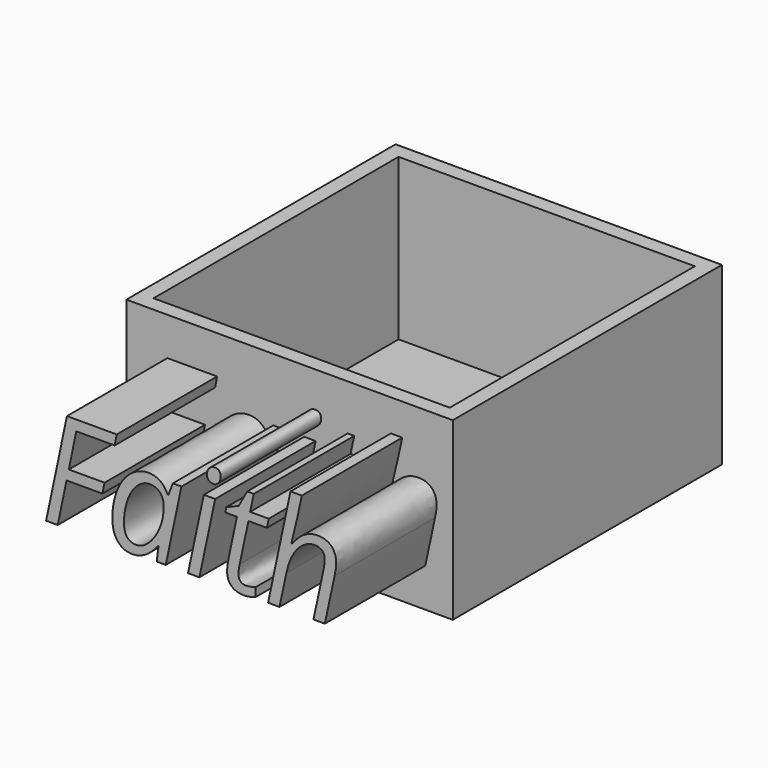
from build123d import *

# Parameters (mm, degrees)
F0_W         = 65
F0_H         = 35
F1_DEPTH     = 67
F2_T         = -3
F3_TEXT_SIZE = 27.6019615639
F4_DEPTH     = 25


# Not quite as in the source:
# - Text() gives the source's letters only with a copy of the font that has no kerning and outlines rounded to 1/6400 em; it was checked with that copy


with BuildPart() as f1:
    # F0 (on Front) → F1 (new body)
    with BuildSketch(Plane.XZ):
        with Locations((-16.7806223035, 12.1302352264)):
            Rectangle(F0_W, F0_H)
    extrude(amount=F1_DEPTH)

    # F2
    f2_openings = [f1.faces().sort_by_distance(p)[0] for p in [
        (-16.780622, -33.5, 29.630235),
    ]]
    offset(amount=F2_T, openings=f2_openings)

    # F3 (on face) → F4 (join)
    with BuildSketch(Plane.XZ.offset(67)):
        with Locations((-46.4393645525, 2.3289155215)):
            Text('Faith', F3_TEXT_SIZE, font='Open Sans', font_style=FontStyle.ITALIC, text_align=(TextAlign.LEFT, TextAlign.BOTTOM))
    extrude(amount=F4_DEPTH)


solid = f1.part
